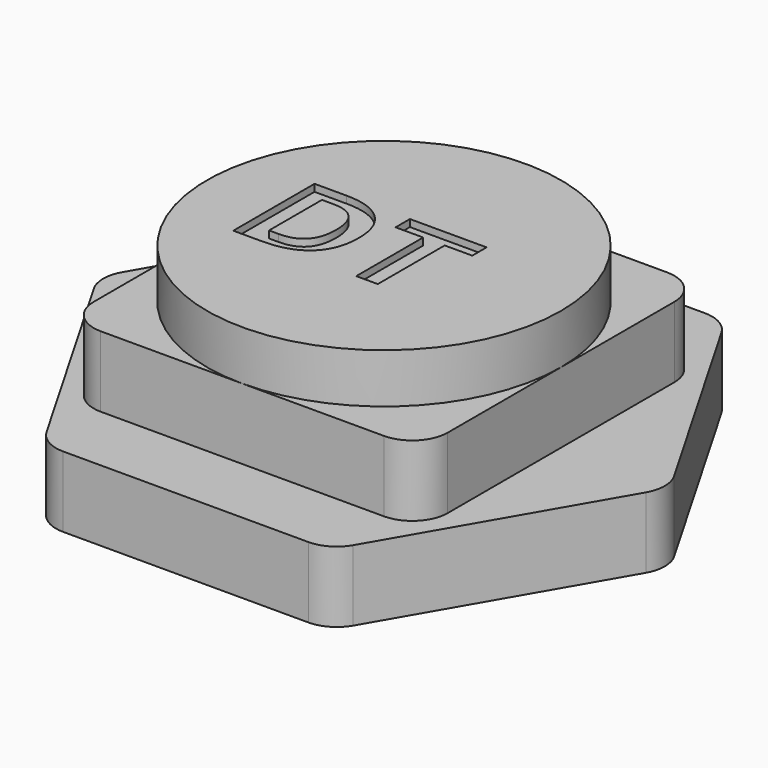
from build123d import *

# Parameters (mm, degrees)
F1_DEPTH     = 10
F2_W         = 50
F2_H         = 50
F3_DEPTH     = 10
F4_R         = 5
F5_R         = 25
F6_DEPTH     = 7
F7_TEXT_SIZE = 20.090637034
F8_DEPTH     = 1


# Not quite as in the source:
# - Text() gives the source's letters only with a copy of the font that has no kerning and outlines rounded to 1/6400 em; it was checked with that copy


with BuildPart() as f1:
    # F0 (on Top) → F1 (new body)
    with BuildSketch(Plane.XY):
        Polygon((20.2072594216, 35), (-20.2072594216, 35), (-40.4145188433, 0), (-20.2072594216, -35), (20.2072594216, -35), (40.4145188433, 0), align=None)
    extrude(amount=F1_DEPTH)

    # F2 (on face) → F3 (join)
    with BuildSketch(Plane.XY.offset(10)):
        Rectangle(F2_W, F2_H)
    extrude(amount=F3_DEPTH)

    # F4
    f4_edges = [f1.edges().sort_by_distance(p)[0] for p in [
        (-40.414519, 0, 5),
        (-20.207259, -35, 5),
        (20.207259, -35, 5),
        (40.414519, 0, 5),
        (20.207259, 35, 5),
        (-20.207259, 35, 5),
        (-25, 25, 15),
        (-25, -25, 15),
        (25, -25, 15),
        (25, 25, 15),
    ]]
    fillet(f4_edges, radius=F4_R)

    # F5 (on face) → F6 (join)
    with BuildSketch(Plane.XY.offset(20)):
        Circle(F5_R)
    extrude(amount=F6_DEPTH)

    # F7 (on face) → F8 (cut)
    with BuildSketch(Plane.XY.offset(27)):
        with Locations((-17, -7.6132937596)):
            Text('DT', F7_TEXT_SIZE, font='Open Sans', font_style=FontStyle.BOLD, text_align=(TextAlign.LEFT, TextAlign.BOTTOM))
    extrude(amount=-F8_DEPTH, mode=Mode.SUBTRACT)


solid = f1.part
